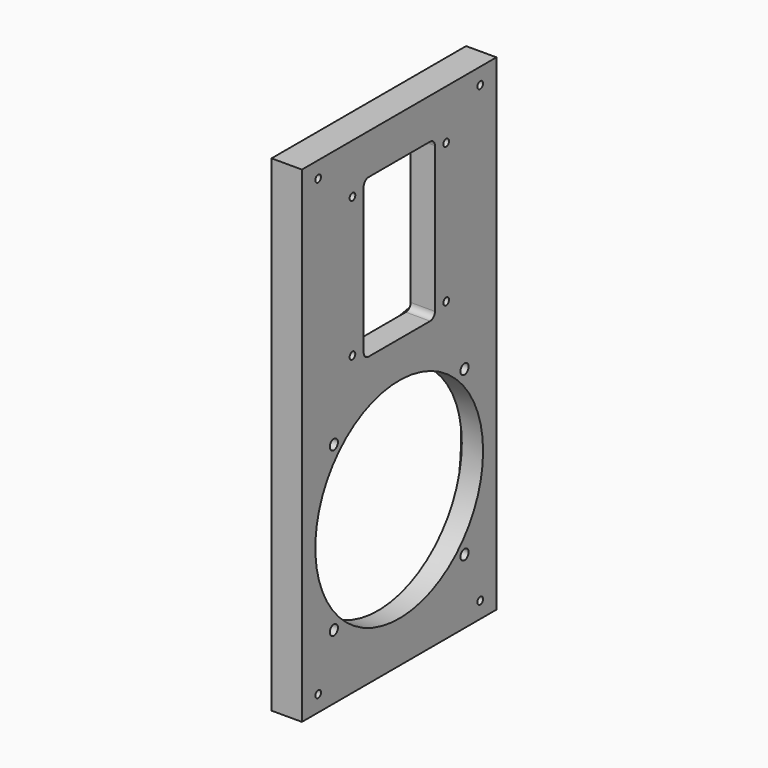
from build123d import *

# Parameters (mm, degrees)
F0_W     = 120
F0_H     = 240
F0_R     = 1.75
F1_DEPTH = 15
F2_DEPTH = 12
F0_R_2   = 2.5
F0_R_3   = 51.75
F3_DEPTH = 10.5


with BuildPart() as f1:
    # F0 (on Right) → F1 (new body)
    with BuildSketch(Plane.YZ):
        with Locations((0, -1.5925480289)):
            Rectangle(F0_W, F0_H)
        with Locations((-49.9999973178, -113.5925480289)):
            Circle(F0_R, mode=Mode.SUBTRACT)
        with BuildLine():
            ThreePointArc((-43.965421423, -1.0136459871), (0, 7.6574519711), (43.965421423, -1.0136459871))
            ThreePointArc((43.965421423, -1.0136459871), (46.5848197582, -2.7577282708), (48.3289020419, -5.377126606))
            ThreePointArc((48.3289020419, -5.377126606), (57, -49.3425480289), (48.3289020419, -93.3079694519))
            ThreePointArc((48.3289020419, -93.3079694519), (46.5848197582, -95.9273677871), (43.965421423, -97.6714500708))
            ThreePointArc((43.965421423, -97.6714500708), (0, -106.3425480289), (-43.965421423, -97.6714500708))
            ThreePointArc((-43.965421423, -97.6714500708), (-46.5848197582, -95.9273677871), (-48.3289020419, -93.3079694519))
            ThreePointArc((-48.3289020419, -93.3079694519), (-57, -49.3425480289), (-48.3289020419, -5.377126606))
            ThreePointArc((-48.3289020419, -5.377126606), (-46.5848197582, -2.7577282708), (-43.965421423, -1.0136459871))
        make_face(mode=Mode.SUBTRACT)
        with Locations((50.0000026822, -113.5925480289)):
            Circle(F0_R, mode=Mode.SUBTRACT)
        with Locations((-49.9999973178, 110.4074519711)):
            Circle(F0_R, mode=Mode.SUBTRACT)
        with BuildLine():
            add(Edge.make_bspline(
                [(32.8620764687, 98.4757185701), (31.4966530962, 98.6776279271), (30.1312297237, 98.8982735514), (28.7658063512, 99.1298205687)],
                knots=[0, 0, 0, 0, 0.0624771081, 0.0624771081, 0.0624771081, 0.0624771081], degree=3))
            add(Edge.make_bspline(
                [(33.6642538877, 94.2964592226), (33.4088016163, 95.6895456718), (33.1411606803, 97.082632121), (32.8620764687, 98.4757185701)],
                knots=[0.9465133763, 0.9465133763, 0.9465133763, 0.9465133763, 1, 1, 1, 1], degree=3))
            add(Edge.make_bspline(
                [(33.6642538877, 24.5184447195), (35.7968030814, 36.1481138033), (38.3630136679, 59.4074519711), (35.7968030814, 82.6667901388), (33.6642538877, 94.2964592226)],
                knots=[0.0534866237, 0.0534866237, 0.0534866237, 0.0534866237, 0.5, 0.9465133763, 0.9465133763, 0.9465133763, 0.9465133763], degree=3))
            add(Edge.make_bspline(
                [(32.8620764687, 20.339185372), (33.1411606803, 21.7322718212), (33.4088016163, 23.1253582703), (33.6642538877, 24.5184447195)],
                knots=[0, 0, 0, 0, 0.0534866237, 0.0534866237, 0.0534866237, 0.0534866237], degree=3))
            add(Edge.make_bspline(
                [(28.7658063512, 19.6850833734), (30.1312297237, 19.9166303908), (31.4966530962, 20.1372760151), (32.8620764687, 20.339185372)],
                knots=[0.9375228919, 0.9375228919, 0.9375228919, 0.9375228919, 1, 1, 1, 1], degree=3))
            add(Edge.make_bspline(
                [(-28.6059896019, 19.6850833734), (-19.0440236097, 18.0635755317), (0.0799083746, 13.7513284104), (19.203840359, 18.0635755317), (28.7658063512, 19.6850833734)],
                knots=[0.0624771081, 0.0624771081, 0.0624771081, 0.0624771081, 0.5, 0.9375228919, 0.9375228919, 0.9375228919, 0.9375228919], degree=3))
            add(Edge.make_bspline(
                [(-32.7022597194, 20.339185372), (-31.3368363469, 20.1372760151), (-29.9714129744, 19.9166303908), (-28.6059896019, 19.6850833734)],
                knots=[0, 0, 0, 0, 0.0624771081, 0.0624771081, 0.0624771081, 0.0624771081], degree=3))
            add(Edge.make_bspline(
                [(-33.5044371384, 24.5184447195), (-33.248984867, 23.1253582703), (-32.981343931, 21.7322718212), (-32.7022597194, 20.339185372)],
                knots=[0.9465133763, 0.9465133763, 0.9465133763, 0.9465133763, 1, 1, 1, 1], degree=3))
            add(Edge.make_bspline(
                [(-33.5044371384, 94.2964592226), (-35.6369863321, 82.6667901388), (-38.2031969186, 59.4074519711), (-35.6369863321, 36.1481138033), (-33.5044371384, 24.5184447195)],
                knots=[0.0534866237, 0.0534866237, 0.0534866237, 0.0534866237, 0.5, 0.9465133763, 0.9465133763, 0.9465133763, 0.9465133763], degree=3))
            add(Edge.make_bspline(
                [(-32.7022597194, 98.4757185701), (-32.981343931, 97.082632121), (-33.248984867, 95.6895456718), (-33.5044371384, 94.2964592226)],
                knots=[0, 0, 0, 0, 0.0534866237, 0.0534866237, 0.0534866237, 0.0534866237], degree=3))
            add(Edge.make_bspline(
                [(-28.6059896019, 99.1298205687), (-29.9714129744, 98.8982735514), (-31.3368363469, 98.6776279271), (-32.7022597194, 98.4757185701)],
                knots=[0.9375228919, 0.9375228919, 0.9375228919, 0.9375228919, 1, 1, 1, 1], degree=3))
            add(Edge.make_bspline(
                [(28.7658063512, 99.1298205687), (19.203840359, 100.7513284104), (0.0799083746, 105.0635755317), (-19.0440236097, 100.7513284104), (-28.6059896019, 99.1298205687)],
                knots=[0.0624771081, 0.0624771081, 0.0624771081, 0.0624771081, 0.5, 0.9375228919, 0.9375228919, 0.9375228919, 0.9375228919], degree=3))
        make_face(mode=Mode.SUBTRACT)
        with Locations((50.0000026822, 110.4074554281)):
            Circle(F0_R, mode=Mode.SUBTRACT)
        with BuildLine():
            add(Edge.make_bspline(
                [(33.6642538877, 94.2964592226), (33.4088016163, 95.6895456718), (33.1411606803, 97.082632121), (32.8620764687, 98.4757185701)],
                knots=[0.9465133763, 0.9465133763, 0.9465133763, 0.9465133763, 1, 1, 1, 1], degree=3))
            add(Edge.make_bspline(
                [(32.8620764687, 98.4757185701), (31.4966530962, 98.6776279271), (30.1312297237, 98.8982735514), (28.7658063512, 99.1298205687)],
                knots=[0, 0, 0, 0, 0.0624771081, 0.0624771081, 0.0624771081, 0.0624771081], degree=3))
            ThreePointArc((28.7658063512, 99.1298205687), (31.9768261624, 97.4851943073), (33.6642538877, 94.2964592226))
        make_face()
        with BuildLine():
            ThreePointArc((-33.5044371384, 94.2964592226), (-31.8170094131, 97.4851943073), (-28.6059896019, 99.1298205687))
            add(Edge.make_bspline(
                [(-28.6059896019, 99.1298205687), (-29.9714129744, 98.8982735514), (-31.3368363469, 98.6776279271), (-32.7022597194, 98.4757185701)],
                knots=[0.9375228919, 0.9375228919, 0.9375228919, 0.9375228919, 1, 1, 1, 1], degree=3))
            add(Edge.make_bspline(
                [(-32.7022597194, 98.4757185701), (-32.981343931, 97.082632121), (-33.248984867, 95.6895456718), (-33.5044371384, 94.2964592226)],
                knots=[0, 0, 0, 0, 0.0534866237, 0.0534866237, 0.0534866237, 0.0534866237], degree=3))
        make_face()
        with BuildLine():
            add(Edge.make_bspline(
                [(32.8620764687, 20.339185372), (33.1411606803, 21.7322718212), (33.4088016163, 23.1253582703), (33.6642538877, 24.5184447195)],
                knots=[0, 0, 0, 0, 0.0534866237, 0.0534866237, 0.0534866237, 0.0534866237], degree=3))
            ThreePointArc((33.6642538877, 24.5184447195), (31.9768261624, 21.3297096348), (28.7658063512, 19.6850833734))
            add(Edge.make_bspline(
                [(28.7658063512, 19.6850833734), (30.1312297237, 19.9166303908), (31.4966530962, 20.1372760151), (32.8620764687, 20.339185372)],
                knots=[0.9375228919, 0.9375228919, 0.9375228919, 0.9375228919, 1, 1, 1, 1], degree=3))
        make_face()
        with BuildLine():
            ThreePointArc((-28.6059896019, 19.6850833734), (-31.8170094131, 21.3297096348), (-33.5044371384, 24.5184447195))
            add(Edge.make_bspline(
                [(-33.5044371384, 24.5184447195), (-33.248984867, 23.1253582703), (-32.981343931, 21.7322718212), (-32.7022597194, 20.339185372)],
                knots=[0.9465133763, 0.9465133763, 0.9465133763, 0.9465133763, 1, 1, 1, 1], degree=3))
            add(Edge.make_bspline(
                [(-32.7022597194, 20.339185372), (-31.3368363469, 20.1372760151), (-29.9714129744, 19.9166303908), (-28.6059896019, 19.6850833734)],
                knots=[0, 0, 0, 0, 0.0624771081, 0.0624771081, 0.0624771081, 0.0624771081], degree=3))
        make_face()
    extrude(amount=-F1_DEPTH)

    # F0 (on Right) → F2 (join)
    with BuildSketch(Plane.YZ):
        with BuildLine():
            add(Edge.make_bspline(
                [(33.6642538877, 94.2964592226), (33.4088016163, 95.6895456718), (33.1411606803, 97.082632121), (32.8620764687, 98.4757185701)],
                knots=[0.9465133763, 0.9465133763, 0.9465133763, 0.9465133763, 1, 1, 1, 1], degree=3))
            add(Edge.make_bspline(
                [(32.8620764687, 98.4757185701), (31.4966530962, 98.6776279271), (30.1312297237, 98.8982735514), (28.7658063512, 99.1298205687)],
                knots=[0, 0, 0, 0, 0.0624771081, 0.0624771081, 0.0624771081, 0.0624771081], degree=3))
            ThreePointArc((28.7658063512, 99.1298205687), (31.9768261624, 97.4851943073), (33.6642538877, 94.2964592226))
        make_face()
        with BuildLine():
            ThreePointArc((33.6642538877, 94.2964592226), (31.9768261624, 97.4851943073), (28.7658063512, 99.1298205687))
            add(Edge.make_bspline(
                [(28.7658063512, 99.1298205687), (19.203840359, 100.7513284104), (0.0799083746, 105.0635755317), (-19.0440236097, 100.7513284104), (-28.6059896019, 99.1298205687)],
                knots=[0.0624771081, 0.0624771081, 0.0624771081, 0.0624771081, 0.5, 0.9375228919, 0.9375228919, 0.9375228919, 0.9375228919], degree=3))
            ThreePointArc((-28.6059896019, 99.1298205687), (-31.8170094131, 97.4851943073), (-33.5044371384, 94.2964592226))
            add(Edge.make_bspline(
                [(-33.5044371384, 94.2964592226), (-35.6369863321, 82.6667901388), (-38.2031969186, 59.4074519711), (-35.6369863321, 36.1481138033), (-33.5044371384, 24.5184447195)],
                knots=[0.0534866237, 0.0534866237, 0.0534866237, 0.0534866237, 0.5, 0.9465133763, 0.9465133763, 0.9465133763, 0.9465133763], degree=3))
            ThreePointArc((-33.5044371384, 24.5184447195), (-31.8170094131, 21.3297096348), (-28.6059896019, 19.6850833734))
            add(Edge.make_bspline(
                [(-28.6059896019, 19.6850833734), (-19.0440236097, 18.0635755317), (0.0799083746, 13.7513284104), (19.203840359, 18.0635755317), (28.7658063512, 19.6850833734)],
                knots=[0.0624771081, 0.0624771081, 0.0624771081, 0.0624771081, 0.5, 0.9375228919, 0.9375228919, 0.9375228919, 0.9375228919], degree=3))
            ThreePointArc((28.7658063512, 19.6850833734), (31.9768261624, 21.3297096348), (33.6642538877, 24.5184447195))
            add(Edge.make_bspline(
                [(33.6642538877, 24.5184447195), (35.7968030814, 36.1481138033), (38.3630136679, 59.4074519711), (35.7968030814, 82.6667901388), (33.6642538877, 94.2964592226)],
                knots=[0.0534866237, 0.0534866237, 0.0534866237, 0.0534866237, 0.5, 0.9465133763, 0.9465133763, 0.9465133763, 0.9465133763], degree=3))
        make_face()
        with Locations((-28.8455340613, 24.9354520307)):
            Circle(F0_R, mode=Mode.SUBTRACT)
        with Locations((-28.8455340613, 93.8794519114)):
            Circle(F0_R, mode=Mode.SUBTRACT)
        with Locations((29.0053508105, 24.9354520307)):
            Circle(F0_R, mode=Mode.SUBTRACT)
        with BuildLine():
            Line((-18.9200916254, 98.4074519711), (19.0799083746, 98.4074519711))
            ThreePointArc((19.0799083746, 98.4074519711), (21.2012287182, 97.5287723146), (22.0799083746, 95.4074519711))
            Line((22.0799083746, 95.4074519711), (22.0799083746, 23.4074519711))
            ThreePointArc((22.0799083746, 23.4074519711), (21.2012287182, 21.2861316275), (19.0799083746, 20.4074519711))
            Line((19.0799083746, 20.4074519711), (-18.9200916254, 20.4074519711))
            ThreePointArc((-18.9200916254, 20.4074519711), (-21.0414119689, 21.2861316275), (-21.9200916254, 23.4074519711))
            Line((-21.9200916254, 23.4074519711), (-21.9200916254, 95.4074519711))
            ThreePointArc((-21.9200916254, 95.4074519711), (-21.0414119689, 97.5287723146), (-18.9200916254, 98.4074519711))
        make_face(mode=Mode.SUBTRACT)
        with Locations((29.0053508105, 93.8794519114)):
            Circle(F0_R, mode=Mode.SUBTRACT)
        with BuildLine():
            ThreePointArc((-33.5044371384, 94.2964592226), (-31.8170094131, 97.4851943073), (-28.6059896019, 99.1298205687))
            add(Edge.make_bspline(
                [(-28.6059896019, 99.1298205687), (-29.9714129744, 98.8982735514), (-31.3368363469, 98.6776279271), (-32.7022597194, 98.4757185701)],
                knots=[0.9375228919, 0.9375228919, 0.9375228919, 0.9375228919, 1, 1, 1, 1], degree=3))
            add(Edge.make_bspline(
                [(-32.7022597194, 98.4757185701), (-32.981343931, 97.082632121), (-33.248984867, 95.6895456718), (-33.5044371384, 94.2964592226)],
                knots=[0, 0, 0, 0, 0.0534866237, 0.0534866237, 0.0534866237, 0.0534866237], degree=3))
        make_face()
    extrude(amount=-F2_DEPTH)

    # F0 (on Right) → F3 (join)
    with BuildSketch(Plane.YZ):
        with BuildLine():
            ThreePointArc((48.3289020419, -5.377126606), (46.5848197582, -2.7577282708), (43.965421423, -1.0136459871))
            ThreePointArc((43.965421423, -1.0136459871), (0, 7.6574519711), (-43.965421423, -1.0136459871))
            ThreePointArc((-43.965421423, -1.0136459871), (-46.5848197582, -2.7577282708), (-48.3289020419, -5.377126606))
            ThreePointArc((-48.3289020419, -5.377126606), (-57, -49.3425480289), (-48.3289020419, -93.3079694519))
            ThreePointArc((-48.3289020419, -93.3079694519), (-46.5848197582, -95.9273677871), (-43.965421423, -97.6714500708))
            ThreePointArc((-43.965421423, -97.6714500708), (0, -106.3425480289), (43.965421423, -97.6714500708))
            ThreePointArc((43.965421423, -97.6714500708), (46.5848197582, -95.9273677871), (48.3289020419, -93.3079694519))
            ThreePointArc((48.3289020419, -93.3079694519), (57, -49.3425480289), (48.3289020419, -5.377126606))
        make_face()
        with Locations((-40.3050865276, -89.6476345566)):
            Circle(F0_R_2, mode=Mode.SUBTRACT)
        with Locations((-40.3050865276, -9.0374615013)):
            Circle(F0_R_2, mode=Mode.SUBTRACT)
        with Locations((40.3050865276, -89.6476345566)):
            Circle(F0_R_2, mode=Mode.SUBTRACT)
        with Locations((0, -49.3425480289)):
            Circle(F0_R_3, mode=Mode.SUBTRACT)
        with Locations((40.3050865276, -9.0374615013)):
            Circle(F0_R_2, mode=Mode.SUBTRACT)
    extrude(amount=-F3_DEPTH)


solid = f1.part
